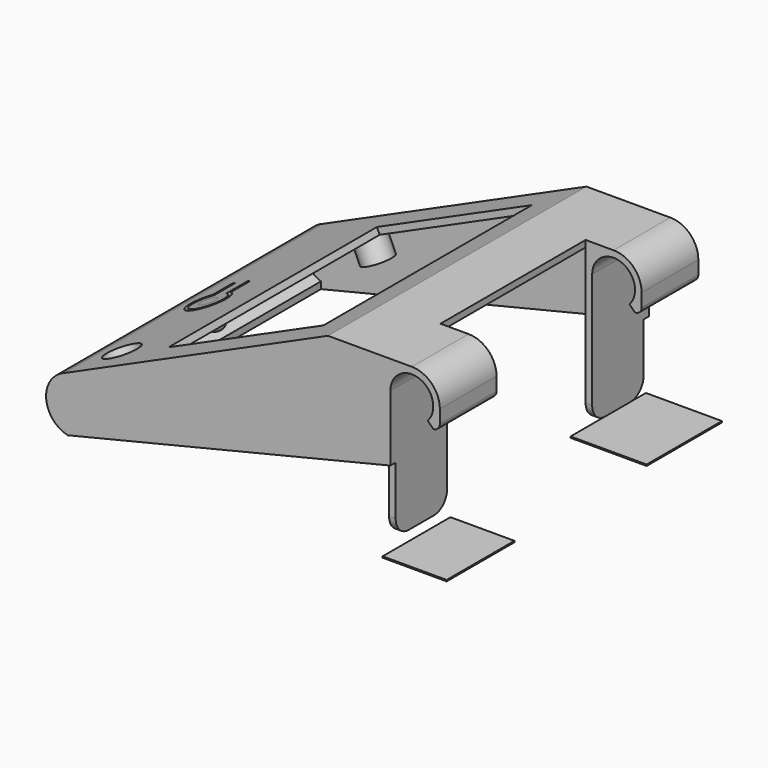
from build123d import *

# Parameters (mm, degrees)
F1_DEPTH  = 49
F2_W      = 51.5
F2_H      = 79
F3_DEPTH  = 2
F2_R      = 1.5
F2_R_2    = 4.5
F4_DEPTH  = 7.3
F6_DEPTH  = 2
F8_DEPTH  = 2
F2_R_3    = 5
F9_DEPTH  = 2
F11_DEPTH = 2
F12_W     = 8.5
F12_H     = 55
F13_DEPTH = 40
F14_R     = 1.99999
F15_W     = 2
F15_H     = 19.5
F16_DEPTH = 20
F17_W     = 2
F17_H     = 19.5
F18_DEPTH = 20
F19_R     = 5
F20_DEPTH = 2
F21_R     = 2.5
F22_DEPTH = 7.5
F23_R     = 2
F25_W     = 23.0630338192
F25_H     = 28.5433605313
F26_DEPTH = 0.4
F25_W_2   = 19.4094888866
F25_H_2   = 25.6890226156


# Not quite as in the source:
# - a fillet or chamfer is up to 0.001 mm smaller than in the source, because OpenCascade refuses the exact size
# - a feature names something its author has since deleted; it is built from what else it names


with BuildPart() as f1:
    # F0 (on Front) → F1 (new body, symmetric)
    with BuildSketch(Plane.XZ):
        with BuildLine():
            Line((-25, 6.5), (-8.5, 6.5))
            Line((-8.5, 6.5), (-8.5, 0))
            Line((-8.5, 0), (-8.5, -20))
            Line((-8.5, -20), (-6.5, -20))
            Line((-6.5, -20), (-6.5, 0))
            ThreePointArc((-6.5, 0), (2.3181097502, 6.072591472), (4.8465745188, -4.3313641539))
            Line((4.8465745188, -4.3313641539), (6.5, -6))
            Line((6.5, -6), (8.5, -6))
            Line((8.5, -6), (8.5, 0))
            ThreePointArc((8.5, 0), (6.0104076401, 6.0104076401), (0, 8.5))
            Line((0, 8.5), (-25.4288327804, 8.5))
            Line((-25.4288327804, 8.5), (-105.428633061, -27.4597649849))
            Line((-105.428633061, -27.4597649849), (-106.3520655314, -27.8748462039))
            ThreePointArc((-106.3520655314, -27.8748462039), (-110.8598066956, -36.4968976222), (-104.3520655314, -43.7293803221))
            Line((-104.3520655314, -43.7293803221), (-104.3520655314, -42.85))
            Line((-104.3520655314, -42.85), (-104.3520655314, -41.6571435378))
            ThreePointArc((-104.3520655314, -41.6571435378), (-108.9268429391, -35.4298576938), (-104.3520655314, -29.2025718498))
            Line((-104.3520655314, -29.2025718498), (-104.3520655314, -29.1686093911))
            Line((-104.3520655314, -29.1686093911), (-25, 6.5))
        make_face()
    extrude(amount=F1_DEPTH, both=True)

    # F2 (on face) → F3 (cut)
    with BuildSketch(Plane(origin=(-6.6328046362, 0, 14.75602097), x_dir=(0.9120927073, 0, 0.409984016), z_dir=(0.409984016, 0, -0.9120927073))):
        with Locations((-55.3874215775, -0.1)):
            Rectangle(F2_W, F2_H)
    extrude(amount=-F3_DEPTH, mode=Mode.SUBTRACT)

    # F2 (on face) → F4 (join)
    with BuildSketch(Plane(origin=(-6.6328046362, 0, 14.75602097), x_dir=(0.9120927073, 0, 0.409984016), z_dir=(0.409984016, 0, -0.9120927073))):
        with BuildLine():
            Line((-20.1374215775, 40.7130369812), (-20.1374215775, 47.9869630188))
            ThreePointArc((-20.1374215775, 47.9869630188), (-27.2874215775, 44.35), (-20.1374215775, 40.7130369812))
        make_face()
        with Locations((-22.7874215775, 44.35)):
            Circle(F2_R, mode=Mode.SUBTRACT)
        with BuildLine():
            Line((-20.1374215775, -47.5869630188), (-20.1374215775, -40.3130369812))
            ThreePointArc((-20.1374215775, -40.3130369812), (-27.2874215775, -43.95), (-20.1374215775, -47.5869630188))
        make_face()
        with Locations((-22.7874215775, -43.95)):
            Circle(F2_R, mode=Mode.SUBTRACT)
        with Locations((-88.7874215775, -43.95)):
            Circle(F2_R_2)
        with Locations((-88.7874215775, -43.95)):
            Circle(F2_R, mode=Mode.SUBTRACT)
        with Locations((-88.7874215775, 44.35)):
            Circle(F2_R_2)
        with Locations((-88.7874215775, 44.35)):
            Circle(F2_R, mode=Mode.SUBTRACT)
    extrude(amount=F4_DEPTH)

    # F5 (on face) → F6 (join)
    with BuildSketch(Plane.XZ.offset(49)):
        with BuildLine():
            Line((-104.3520655314, -43.7293803221), (-6.5, -20))
            Line((-6.5, -20), (-8.5, -20))
            Line((-8.5, -20), (-8.5, 6.5))
            Line((-8.5, 6.5), (-25, 6.5))
            Line((-25, 6.5), (-104.3520655314, -29.1686093911))
            Line((-104.3520655314, -29.1686093911), (-104.3520655314, -29.2025718498))
            ThreePointArc((-104.3520655314, -29.2025718498), (-108.9268429391, -35.4298576938), (-104.3520655314, -41.6571435378))
            Line((-104.3520655314, -41.6571435378), (-104.3520655314, -43.7293803221))
        make_face()
    extrude(amount=-F6_DEPTH)

    # F7 (on face) → F8 (join)
    with BuildSketch(Plane(origin=(0, 49, 0), x_dir=(-1, 0, 0), z_dir=(0, 1, 0))):
        with BuildLine():
            Line((8.5, -20), (6.5, -20))
            Line((6.5, -20), (104.3520655314, -43.7293803221))
            Line((104.3520655314, -43.7293803221), (104.3520655314, -41.6571435378))
            ThreePointArc((104.3520655314, -41.6571435378), (108.9268429391, -35.4298576938), (104.3520655314, -29.2025718498))
            Line((104.3520655314, -29.2025718498), (104.3520655314, -29.1686093911))
            Line((104.3520655314, -29.1686093911), (25, 6.5))
            Line((25, 6.5), (8.5, 6.5))
            Line((8.5, 6.5), (8.5, -20))
        make_face()
    extrude(amount=-F8_DEPTH)

    # F2 (on face) → F9 (cut)
    with BuildSketch(Plane(origin=(-6.6328046362, 0, 14.75602097), x_dir=(0.9120927073, 0, 0.409984016), z_dir=(0.409984016, 0, -0.9120927073))):
        with Locations((-98.7513456427, 37)):
            Circle(F2_R_3)
    extrude(amount=-F9_DEPTH, mode=Mode.SUBTRACT)

    # F10 (on face) → F11 (cut)
    with BuildSketch(Plane(origin=(0, 49, 0), x_dir=(-1, 0, 0), z_dir=(0, 1, 0))):
        Polygon((63.2235160953, -24.4957862935), (39.5091057066, -13.8362018777), (38.0741616506, -17.0285263531), (61.7885720393, -27.6881107689), align=None)
    extrude(amount=-F11_DEPTH, mode=Mode.SUBTRACT)

    # F12 (on face) → F13 (cut)
    with BuildSketch(Plane.XY.offset(8.5)):
        with Locations((4.25, 0)):
            Rectangle(F12_W, F12_H)
        with Locations((-4.25, 0)):
            Rectangle(F12_W, F12_H)
    extrude(amount=-F13_DEPTH, mode=Mode.SUBTRACT)

    # F14 (radius 2 in the source; OpenCascade refuses exactly that, so slightly less here)
    f14_edges = [f1.edges().sort_by_distance(p)[0] for p in [
        (8.5, 38.25, -6),
        (8.5, -38.25, -6),
    ]]
    fillet(f14_edges, radius=F14_R)

    # F15 (on face) → F16 (join)
    with BuildSketch(Plane(origin=(0, 0, -20), x_dir=(1, 0, 0), z_dir=(0, 0, -1))):
        with Locations((-7.5, 37.25)):
            Rectangle(F15_W, F15_H)
    extrude(amount=F16_DEPTH)

    # F17 (on face) → F18 (join)
    with BuildSketch(Plane(origin=(0, 0, -20), x_dir=(1, 0, 0), z_dir=(0, 0, -1))):
        with Locations((-7.5, -37.25)):
            Rectangle(F17_W, F17_H)
    extrude(amount=F18_DEPTH)

    # F19
    f19_edges = [f1.edges().sort_by_distance(p)[0] for p in [
        (-7.5, 47, -40),
        (-7.5, 27.5, -40),
        (-7.5, -27.5, -40),
        (-7.5, -47, -40),
    ]]
    fillet(f19_edges, radius=F19_R)

    # F2 (on face) → F20 (cut)
    with BuildSketch(Plane(origin=(-6.6328046362, 0, 14.75602097), x_dir=(0.9120927073, 0, 0.409984016), z_dir=(0.409984016, 0, -0.9120927073))):
        with BuildLine():
            ThreePointArc((-100.7513456427, -0.282575695), (-98.7513456427, 9.3), (-96.7513456427, -0.282575695))
            Line((-96.7513456427, -0.282575695), (-96.7513456427, -8.282575695))
            Line((-96.7513456427, -8.282575695), (-95.7513456427, -8.282575695))
            Line((-95.7513456427, -8.282575695), (-95.7513456427, -0.8961524227))
            ThreePointArc((-95.7513456427, -0.8961524227), (-98.7513456427, 10.3), (-101.7513456427, -0.8961524227))
            Line((-101.7513456427, -0.8961524227), (-101.7513456427, -8.282575695))
            Line((-101.7513456427, -8.282575695), (-100.7513456427, -8.282575695))
            Line((-100.7513456427, -8.282575695), (-100.7513456427, -0.282575695))
        make_face()
    extrude(amount=-F20_DEPTH, mode=Mode.SUBTRACT)

    # F21 (on face) → F22 (join)
    with BuildSketch(Plane(origin=(-7.4527726682, 0, 16.5802063845), x_dir=(0.9120927073, 0, 0.409984016), z_dir=(-0.409984016, 0, 0.9120927073))):
        with Locations((-98.7513456427, -4.3)):
            Circle(F21_R)
    extrude(amount=-F22_DEPTH)

    # F23
    f23_edges = [f1.edges().sort_by_distance(p)[0] for p in [
        (-96.728507, -4.3, -31.771922),
    ]]
    fillet(f23_edges, radius=F23_R)


with BuildPart() as f1_1:
    # F24: moved
    add(f1.part.moved(Location((53.5, 0, 43.8))))


with BuildPart() as f26:
    # F25 (on Top) → F26 (new body)
    with BuildSketch(Plane.XY):
        with Locations((54.4244498014, 38.7197062373)):
            Rectangle(F25_W, F25_H)
    extrude(amount=F26_DEPTH)


with BuildPart() as f26b:
    # F25 (on Top) → F26, piece 2 (new body)
    with BuildSketch(Plane.XY):
        with Locations((56.2512222677, -38.5186253116)):
            Rectangle(F25_W_2, F25_H_2)
    extrude(amount=F26_DEPTH)


solid = Compound([f1_1.part, f26.part, f26b.part])
